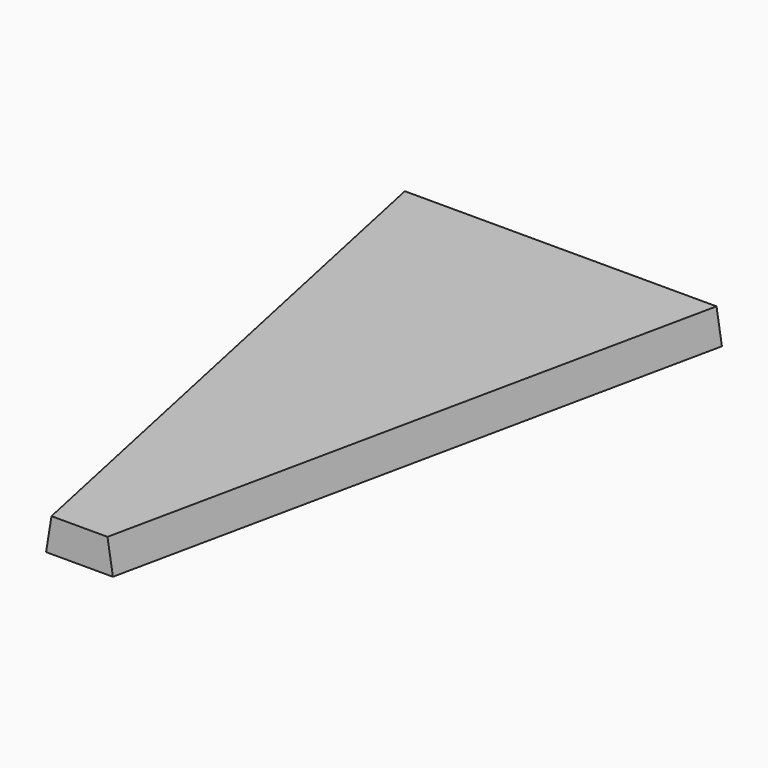
from build123d import *

# Parameters (mm, degrees)
F2_DEPTH   = 25.4
F3_SIZE2   = 4.022955
F3_SIZE    = 25.39999
F3_2_SIZE2 = 4.022955
F3_2_SIZE  = 25.39999


# Not quite as in the source:
# - a fillet or chamfer is up to 0.001 mm smaller than in the source, because OpenCascade refuses the exact size


with BuildPart() as f2:
    # F1 (on Top) → F2 (new body)
    with BuildSketch(Plane.XY):
        Polygon((-122.5808599955, 457.2), (-25.4, 0), (25.4, 0), (122.5808599955, 457.2), align=None)
    extrude(amount=F2_DEPTH)

    # F3 (size 25.4 and 4.0229647842 in the source; OpenCascade refuses exactly that, so slightly less here)
    f3_edges = [f2.edges().sort_by_distance(p)[0] for p in [
        (-73.99043, 228.6, 25.4),
    ]]
    f3_side = f2.faces().sort_by_distance((-73.99043, 228.6, 12.7))[0]
    chamfer(f3_edges, length=F3_SIZE, length2=F3_SIZE2, reference=f3_side)

    # F3#2 (size 25.4 and 4.0229647842 in the source; OpenCascade refuses exactly that, so slightly less here)
    f3_2_edges = [f2.edges().sort_by_distance(p)[0] for p in [
        (73.99043, 228.6, 25.4),
    ]]
    f3_2_side = f2.faces().sort_by_distance((73.99043, 228.6, 12.7))[0]
    chamfer(f3_2_edges, length=F3_2_SIZE, length2=F3_2_SIZE2, reference=f3_2_side)


solid = f2.part
